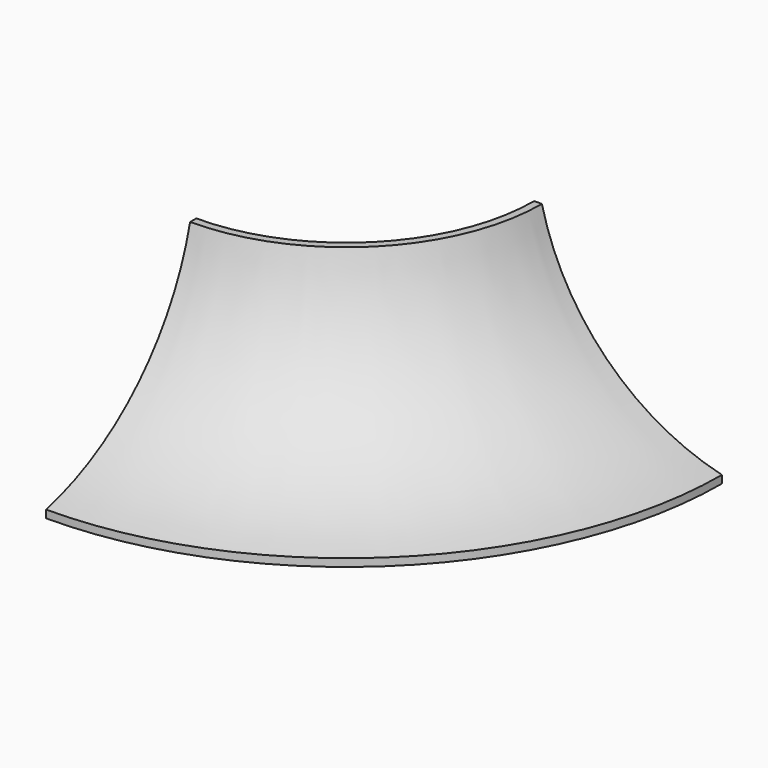
from build123d import *

# Parameters (mm, degrees)
F4_ANGLE = 90


# Not quite as in the source:
# - a feature names something its author has since deleted; it is built from what else it names


with BuildPart() as f4:
    # F1 (on Right) → F4 (revolve)
    with BuildSketch(Plane.YZ):
        with BuildLine():
            Line((-50, 2.0555875069), (-50, 0))
            ThreePointArc((-50, 0), (-35.3898801458, 5.2614268959), (-22.3833982704, 13.7449193584))
            ThreePointArc((-22.3833982704, 13.7449193584), (-21.6521933869, 14.3623617736), (-20.9298823871, 14.9901854251))
            ThreePointArc((-20.9298823871, 14.9901854251), (-19.3758122064, 16.40450242), (-17.8668574762, 17.8668574762))
            ThreePointArc((-17.8668574762, 17.8668574762), (-16.40450242, 19.3758122064), (-14.9901854251, 20.9298823871))
            ThreePointArc((-14.9901854251, 20.9298823871), (-14.3623617736, 21.6521933869), (-13.7449193584, 22.3833982704))
            ThreePointArc((-13.7449193584, 22.3833982704), (-5.2614268959, 35.3898801458), (0, 50))
            Line((0, 50), (-2.0555875069, 50))
            ThreePointArc((-2.0555875069, 50), (-19.2810710386, 19.2810710386), (-50, 2.0555875069))
        make_face()
        with BuildLine():
            ThreePointArc((-20.9298823871, 14.9901854251), (-21.6521933869, 14.3623617736), (-22.3833982704, 13.7449193584))
            Line((-22.3833982704, 13.7449193584), (-15.1433829629, 6.5049040509))
            Line((-15.1433829629, 6.5049040509), (-12.4446010129, 6.5049040509))
            Line((-12.4446010129, 6.5049040509), (-20.9298823871, 14.9901854251))
        make_face()
        with BuildLine():
            ThreePointArc((-13.7449193584, 22.3833982704), (-14.3623617736, 21.6521933869), (-14.9901854251, 20.9298823871))
            Line((-14.9901854251, 20.9298823871), (-6.5049040509, 12.4446010129))
            Line((-6.5049040509, 12.4446010129), (-6.5049040509, 15.1433829629))
            Line((-6.5049040509, 15.1433829629), (-13.7449193584, 22.3833982704))
        make_face()
    revolve(axis=Axis((0, 50, 28.3559039235), (0, 0, 1)), revolution_arc=F4_ANGLE)


solid = f4.part
